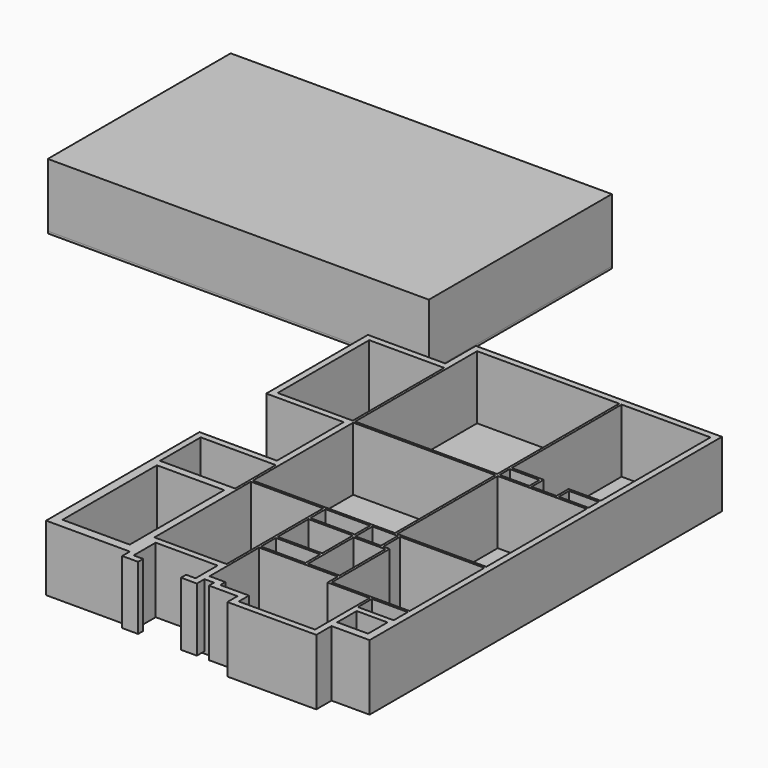
from build123d import *

# Parameters (mm, degrees)
F2_DEPTH = 101.6
F0_W     = 6096
F0_H     = 10972.8
F0_W_2   = 9144
F0_W_3   = 3048
F0_W_4   = 3600.45
F0_H_2   = 5486.4
F0_W_5   = 3225.8
F0_H_3   = 5664.2
F0_W_6   = 114.3
F0_H_4   = 6019.8
F0_H_5   = 609.6
F0_W_7   = 1422.4
F0_H_6   = 114.3
F0_W_8   = 1193.8
F0_H_7   = 76.2
F0_H_8   = 863.6
F0_W_9   = 254
F0_W_10  = 1219.2
F0_H_9   = 844.55
F0_W_11  = 1479.55
F0_H_10  = 1168.4
F3_DEPTH = 3048


with BuildPart() as f2:
    # F1 (on Top) → F2 (new body)
    with BuildSketch(Plane.XY):
        Polygon((3714.75, -11931.65), (0, -11931.65), (0, -21132.8), (4324.35, -21132.8), (4324.35, -19964.4), (7296.15, -19964.4), (7296.15, -21132.8), (8058.15, -21132.8), (8058.15, -21437.6), (9429.75, -21437.6), (9429.75, -22047.2), (13696.95, -22047.2), (13696.95, -21132.8), (15525.75, -21132.8), (15525.75, 0), (3714.75, 0), (3714.75, -1828.8), (0, -1828.8), (0, -7924.8), (3714.75, -7924.8), align=None)
    extrude(amount=-F2_DEPTH)

    # F0 (on Top) → F3 (join)
    with BuildSketch(Plane.XY):
        Polygon((15525.75, 0), (3714.75, 0), (3714.75, -1828.8), (0, -1828.8), (0, -7924.8), (3714.75, -7924.8), (3714.75, -11931.65), (0, -11931.65), (0, -14674.85), (304.8, -14674.85), (304.8, -12236.45), (3905.25, -12236.45), (3905.25, -14674.85), (4019.55, -14674.85), (4019.55, -13868.4), (4019.55, -13754.1), (4019.55, -7734.3), (4019.55, -7620), (4019.55, -304.8), (10839.45, -304.8), (10953.75, -304.8), (15220.95, -304.8), (15220.95, -6896.1), (15220.95, -7010.4), (15220.95, -7620), (15220.95, -7734.3), (15220.95, -13754.1), (15220.95, -13868.4), (15220.95, -18351.5), (15220.95, -18465.8), (15220.95, -19310.35), (15430.5, -19310.35), (15430.5, -21037.55), (13392.15, -21037.55), (13392.15, -21742.4), (9734.55, -21742.4), (9734.55, -21132.8), (8362.95, -21132.8), (8362.95, -20828), (7600.95, -20828), (7600.95, -19659.6), (7486.65, -19659.6), (4019.55, -19659.6), (4019.55, -21132.8), (4019.55, -21590), (4781.55, -21590), (4781.55, -21285.2), (4324.35, -21285.2), (4324.35, -19964.4), (7296.15, -19964.4), (7296.15, -21285.2), (6838.95, -21285.2), (6838.95, -21590), (7600.95, -21590), (7600.95, -21132.8), (8058.15, -21132.8), (8058.15, -21437.6), (9429.75, -21437.6), (9429.75, -22047.2), (13696.95, -22047.2), (13696.95, -21132.8), (15525.75, -21132.8), align=None)
        with Locations((2105.025, -4876.8)):
            Rectangle(F0_W_4, F0_H_2, mode=Mode.SUBTRACT)
        Polygon((304.8, -14674.85), (0, -14674.85), (0, -21132.8), (4019.55, -21132.8), (4019.55, -19659.6), (4019.55, -14674.85), (3905.25, -14674.85), align=None)
        with Locations((2051.05, -17862.55)):
            Rectangle(F0_W_5, F0_H_3, mode=Mode.SUBTRACT)
        Polygon((10839.45, -304.8), (10839.45, -7620), (10953.75, -7620), (10953.75, -7010.4), (10953.75, -6896.1), (10953.75, -304.8), align=None)
        Polygon((4019.55, -7620), (4019.55, -7734.3), (10839.45, -7734.3), (10953.75, -7734.3), (12376.15, -7734.3), (12376.15, -7620), (10953.75, -7620), (10839.45, -7620), align=None)
        with Locations((10896.6, -10744.2)):
            Rectangle(F0_W_6, F0_H_4)
        with Locations((12433.3, -7315.2)):
            Rectangle(F0_W_6, F0_H_5)
        with Locations((11664.95, -6953.25)):
            Rectangle(F0_W_7, F0_H_6)
        with Locations((12433.3, -6953.25)):
            Rectangle(F0_W_6, F0_H_6)
        with Locations((12433.3, -7677.15)):
            Rectangle(F0_W_6, F0_H_6)
        with Locations((13087.35, -7677.15)):
            Rectangle(F0_W_8, F0_H_6)
        with Locations((14509.75, -6953.25)):
            Rectangle(F0_W_7, F0_H_6)
        with Locations((13741.4, -6953.25)):
            Rectangle(F0_W_6, F0_H_6)
        with Locations((13741.4, -7315.2)):
            Rectangle(F0_W_6, F0_H_5)
        with Locations((13741.4, -7677.15)):
            Rectangle(F0_W_6, F0_H_6)
        with Locations((14509.75, -7677.15)):
            Rectangle(F0_W_7, F0_H_6)
        Polygon((10839.45, -13754.1), (9848.85, -13754.1), (9848.85, -13868.4), (11068.05, -13868.4), (11182.35, -13868.4), (15220.95, -13868.4), (15220.95, -13754.1), (10953.75, -13754.1), align=None)
        with Locations((11125.2, -13906.5)):
            Rectangle(F0_W_6, F0_H_7)
        with Locations((11125.2, -14846.3)):
            Rectangle(F0_W_6, F0_H_7)
        with Locations((11125.2, -14376.4)):
            Rectangle(F0_W_6, F0_H_8)
        Polygon((11372.85, -17741.9), (11372.85, -17856.2), (11487.15, -17856.2), (11487.15, -14884.4), (11182.35, -14884.4), (11068.05, -14884.4), (9848.85, -14884.4), (9848.85, -14998.7), (10763.25, -14998.7), (11372.85, -14998.7), (11372.85, -16217.9), (11372.85, -16929.1), align=None)
        Polygon((4019.55, -13754.1), (4019.55, -13868.4), (7486.65, -13868.4), (7600.95, -13868.4), (8515.35, -13868.4), (9734.55, -13868.4), (9848.85, -13868.4), (9848.85, -13754.1), align=None)
        Polygon((7486.65, -13868.4), (7486.65, -19659.6), (7600.95, -19659.6), (7600.95, -17856.2), (7600.95, -17741.9), (7600.95, -16852.9), (7600.95, -16738.6), (7600.95, -14897.1), (7600.95, -14782.8), (7600.95, -13868.4), align=None)
        Polygon((8515.35, -14782.8), (7600.95, -14782.8), (7600.95, -14897.1), (9124.95, -14897.1), (9734.55, -14897.1), (9734.55, -14782.8), align=None)
        Polygon((7600.95, -16738.6), (7600.95, -16852.9), (9734.55, -16852.9), (9734.55, -16738.6), (9124.95, -16738.6), align=None)
        Polygon((7600.95, -17741.9), (7600.95, -17856.2), (11372.85, -17856.2), (11372.85, -17741.9), (9848.85, -17741.9), (9734.55, -17741.9), align=None)
        Polygon((9848.85, -14884.4), (9848.85, -13868.4), (9734.55, -13868.4), (9734.55, -14782.8), (9734.55, -14897.1), (9734.55, -16738.6), (9734.55, -16852.9), (9734.55, -17741.9), (9848.85, -17741.9), (9848.85, -16929.1), (9848.85, -14998.7), align=None)
        Polygon((11487.15, -17856.2), (11372.85, -17856.2), (11372.85, -18465.8), (13392.15, -18465.8), (13506.45, -18465.8), (13747.75, -18465.8), (13747.75, -18351.5), (11487.15, -18351.5), align=None)
        with Locations((15093.95, -18408.65)):
            Rectangle(F0_W_9, F0_H_6)
        with Locations((14357.35, -18408.65)):
            Rectangle(F0_W_10, F0_H_6)
        with Locations((13449.3, -18888.075)):
            Rectangle(F0_W_6, F0_H_9)
        Polygon((13506.45, -19310.35), (13392.15, -19310.35), (13392.15, -21037.55), (15430.5, -21037.55), (15430.5, -19310.35), (15220.95, -19310.35), align=None)
        with Locations((14411.325, -20173.95)):
            Rectangle(F0_W_11, F0_H_10, mode=Mode.SUBTRACT)
    extrude(amount=F3_DEPTH)


with BuildPart() as f2b:
    # F0 (on Top) → F2, piece 2 (new body)
    with BuildSketch(Plane.XY):
        with Locations((-15240, 7315.2)):
            Rectangle(F0_W, F0_H)
        with Locations((-7620, 7315.2)):
            Rectangle(F0_W_2, F0_H)
        with Locations((-1524, 7315.2)):
            Rectangle(F0_W_3, F0_H)
    extrude(amount=-F2_DEPTH)


with BuildPart() as f3:
    # F0 (on Top) → F3, piece 2 (new body)
    with BuildSketch(Plane.XY):
        with Locations((-7620, 7315.2)):
            Rectangle(F0_W_2, F0_H)
        with Locations((-1524, 7315.2)):
            Rectangle(F0_W_3, F0_H)
        with Locations((-15240, 7315.2)):
            Rectangle(F0_W, F0_H)
    extrude(amount=F3_DEPTH)


solid = Compound([f2.part, f2b.part, f3.part])
